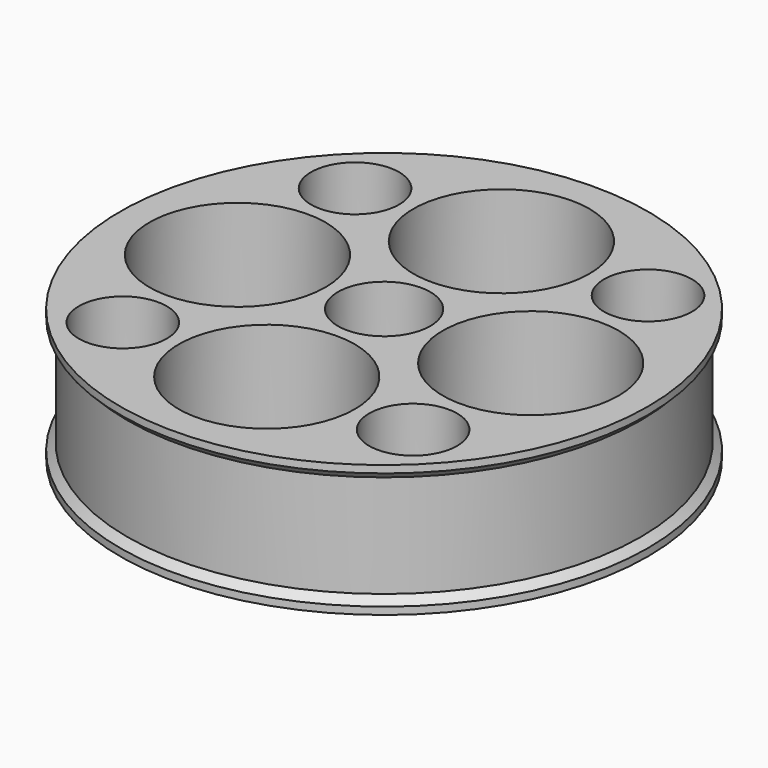
from build123d import *

# Parameters (mm, degrees)
F0_R     = 17.5
F0_R_2   = 3
F0_R_3   = 6
F0_R_4   = 3.15
F1_DEPTH = 7
F2_R     = 18
F2_R_2   = 17.5
F2_R_3   = 3
F2_R_4   = 6
F2_R_5   = 3.15
F3_DEPTH = 1
F4_R     = 18
F4_R_2   = 17.5
F4_R_3   = 3
F4_R_4   = 6
F4_R_5   = 3.15
F5_DEPTH = 1
F6_SIZE  = 0.49999


# Not quite as in the source:
# - a fillet or chamfer is up to 0.001 mm smaller than in the source, because OpenCascade refuses the exact size


with BuildPart() as f1:
    # F0 (on Top) → F1 (new body)
    with BuildSketch(Plane.XY):
        Circle(F0_R)
        with Locations((-9.8994949366, -9.8994949366)):
            Circle(F0_R_2, mode=Mode.SUBTRACT)
        with Locations((0, -10)):
            Circle(F0_R_3, mode=Mode.SUBTRACT)
        with Locations((9.8994949366, -9.8994949366)):
            Circle(F0_R_2, mode=Mode.SUBTRACT)
        with Locations((-10, 0)):
            Circle(F0_R_3, mode=Mode.SUBTRACT)
        with Locations((-9.8994949366, 9.8994949366)):
            Circle(F0_R_2, mode=Mode.SUBTRACT)
        Circle(F0_R_4, mode=Mode.SUBTRACT)
        with Locations((10, 0)):
            Circle(F0_R_3, mode=Mode.SUBTRACT)
        with Locations((0, 10)):
            Circle(F0_R_3, mode=Mode.SUBTRACT)
        with Locations((10, 10)):
            Circle(F0_R_2, mode=Mode.SUBTRACT)
    extrude(amount=F1_DEPTH)

    # F2 (on face) → F3 (join)
    with BuildSketch(Plane.XY.offset(7)):
        Circle(F2_R)
        Circle(F2_R_2, mode=Mode.SUBTRACT)
        Circle(F2_R_2)
        with Locations((-9.8994949366, -9.8994949366)):
            Circle(F2_R_3, mode=Mode.SUBTRACT)
        with Locations((0, -10)):
            Circle(F2_R_4, mode=Mode.SUBTRACT)
        with Locations((9.8994949366, -9.8994949366)):
            Circle(F2_R_3, mode=Mode.SUBTRACT)
        with Locations((-10, 0)):
            Circle(F2_R_4, mode=Mode.SUBTRACT)
        with Locations((-9.8994949366, 9.8994949366)):
            Circle(F2_R_3, mode=Mode.SUBTRACT)
        Circle(F2_R_5, mode=Mode.SUBTRACT)
        with Locations((10, 0)):
            Circle(F2_R_4, mode=Mode.SUBTRACT)
        with Locations((0, 10)):
            Circle(F2_R_4, mode=Mode.SUBTRACT)
        with Locations((10, 10)):
            Circle(F2_R_3, mode=Mode.SUBTRACT)
    extrude(amount=F3_DEPTH)

    # F4 (on face) → F5 (join)
    with BuildSketch(Plane(origin=(0, 0, 0), x_dir=(1, 0, 0), z_dir=(0, 0, -1))):
        Circle(F4_R)
        Circle(F4_R_2, mode=Mode.SUBTRACT)
        Circle(F4_R_2)
        with Locations((-9.8994949366, -9.8994949366)):
            Circle(F4_R_3, mode=Mode.SUBTRACT)
        with Locations((0, -10)):
            Circle(F4_R_4, mode=Mode.SUBTRACT)
        with Locations((10, -10)):
            Circle(F4_R_3, mode=Mode.SUBTRACT)
        with Locations((-10, 0)):
            Circle(F4_R_4, mode=Mode.SUBTRACT)
        with Locations((-9.8994949366, 9.8994949366)):
            Circle(F4_R_3, mode=Mode.SUBTRACT)
        Circle(F4_R_5, mode=Mode.SUBTRACT)
        with Locations((10, 0)):
            Circle(F4_R_4, mode=Mode.SUBTRACT)
        with Locations((0, 10)):
            Circle(F4_R_4, mode=Mode.SUBTRACT)
        with Locations((9.8994949366, 9.8994949366)):
            Circle(F4_R_3, mode=Mode.SUBTRACT)
    extrude(amount=F5_DEPTH)

    # F6 (size 0.5 in the source; OpenCascade refuses exactly that, so slightly less here)
    f6_edges = [f1.edges().sort_by_distance(p)[0] for p in [
        (-18, 0, 0),
        (-18, 0, 7),
    ]]
    chamfer(f6_edges, length=F6_SIZE)


solid = f1.part
